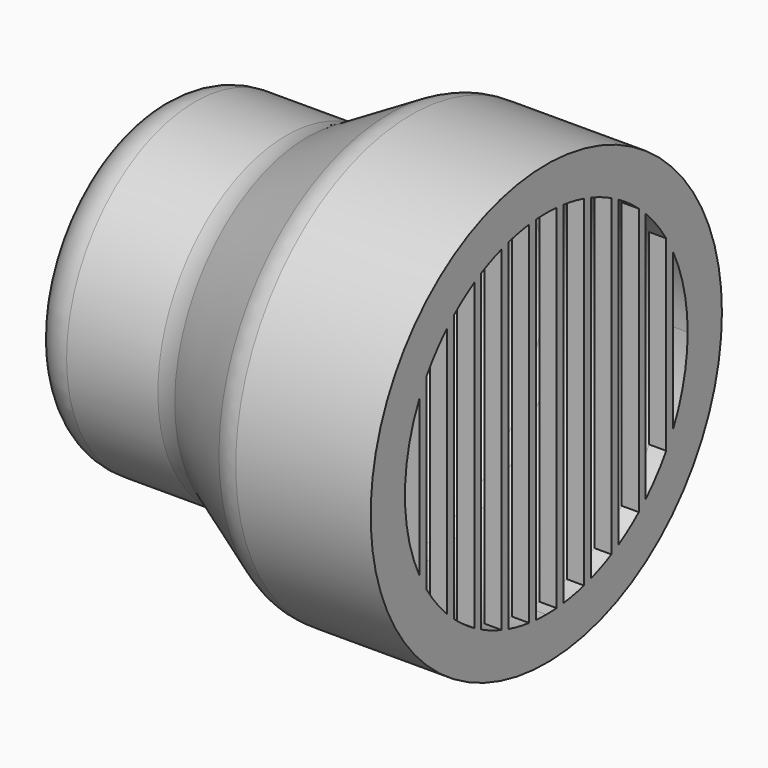
from build123d import *

# Parameters (mm, degrees)
F2_R     = 25.625
F3_DEPTH = 2
F5_DEPTH = 2
F6_R     = 4.99999
F7_R     = 3


# Not quite as in the source:
# - a fillet or chamfer is up to 0.001 mm smaller than in the source, because OpenCascade refuses the exact size


with BuildPart() as f1:
    # F0 (on Top) → F1 (revolve)
    with BuildSketch(Plane.XY):
        Polygon((-18.3333333333, 18.75), (-18.3333333333, 13.75), (0, 13.75), (11.907849302, 20.625), (25.657849302, 20.625), (25.657849302, 25.625), (10.5681033399, 25.625), (-1.3397459622, 18.75), align=None)
    revolve(axis=Axis((-8.7595172226, 0, 0), (1, 0, 0)))

    # F2 (on face) → F3 (join)
    with BuildSketch(Plane.YZ.offset(25.657849302)):
        Circle(F2_R)
    extrude(amount=F3_DEPTH)

    # F4 (on face) → F5 (cut, through all)
    with BuildSketch(Plane.YZ.offset(27.657849302)):
        with BuildLine():
            ThreePointArc((20.625, 0), (20.0867260274, 4.6812458278), (18.5, 9.1181481124))
            Line((18.5, 9.1181481124), (18.5, -9.1181481124))
            ThreePointArc((18.5, -9.1181481124), (20.0867260274, -4.6812458278), (20.625, 0))
        make_face()
        with BuildLine():
            ThreePointArc((17.5, 10.9151557479), (16.1096351924, 12.8790635905), (14.5, 14.6676727875))
            Line((14.5, 14.6676727875), (14.5, -14.6676727875))
            ThreePointArc((14.5, -14.6676727875), (16.1096351924, -12.8790635905), (17.5, -10.9151557479))
            Line((17.5, -10.9151557479), (17.5, 10.9151557479))
        make_face()
        with BuildLine():
            ThreePointArc((13.5, 15.5929671647), (12.0484676296, 16.7399239179), (10.5, 17.7522005678))
            Line((10.5, 17.7522005678), (10.5, -17.7522005678))
            ThreePointArc((10.5, -17.7522005678), (12.0484676296, -16.7399239179), (13.5, -15.5929671647))
            Line((13.5, -15.5929671647), (13.5, 15.5929671647))
        make_face()
        with BuildLine():
            ThreePointArc((9.5, 18.3068463969), (8.0250486473, 18.9997162929), (6.5, 19.573978262))
            Line((6.5, 19.573978262), (6.5, -19.573978262))
            ThreePointArc((6.5, -19.573978262), (8.0250486473, -18.9997162929), (9.5, -18.3068463969))
            Line((9.5, -18.3068463969), (9.5, 18.3068463969))
        make_face()
        with BuildLine():
            ThreePointArc((5.5, 19.8781444054), (4.0110398588, 20.2312180615), (2.5, 20.4729241927))
            Line((2.5, 20.4729241927), (2.5, -20.4729241927))
            ThreePointArc((2.5, -20.4729241927), (4.0110398588, -20.2312180615), (5.5, -19.8781444054))
            Line((5.5, -19.8781444054), (5.5, 19.8781444054))
        make_face()
        with BuildLine():
            ThreePointArc((1.5, 20.5703822279), (0.7504970188, 20.6113410341), (0, 20.625))
            ThreePointArc((0, 20.625), (-0.7504970188, 20.6113410341), (-1.5, 20.5703822279))
            Line((-1.5, 20.5703822279), (-1.5, -20.5703822279))
            ThreePointArc((-1.5, -20.5703822279), (-0.7504970188, -20.6113410341), (0, -20.625))
            ThreePointArc((0, -20.625), (0.7504970188, -20.6113410341), (1.5, -20.5703822279))
            Line((1.5, -20.5703822279), (1.5, 20.5703822279))
        make_face()
        with BuildLine():
            Line((-2.5, -20.4729241927), (-2.5, 20.4729241927))
            ThreePointArc((-2.5, 20.4729241927), (-4.0110398588, 20.2312180615), (-5.5, 19.8781444054))
            Line((-5.5, 19.8781444054), (-5.5, -19.8781444054))
            ThreePointArc((-5.5, -19.8781444054), (-4.0110398588, -20.2312180615), (-2.5, -20.4729241927))
        make_face()
        with BuildLine():
            Line((-6.5, -19.573978262), (-6.5, 19.573978262))
            ThreePointArc((-6.5, 19.573978262), (-8.0250486473, 18.9997162929), (-9.5, 18.3068463969))
            Line((-9.5, 18.3068463969), (-9.5, -18.3068463969))
            ThreePointArc((-9.5, -18.3068463969), (-8.0250486473, -18.9997162929), (-6.5, -19.573978262))
        make_face()
        with BuildLine():
            Line((-10.5, -17.7522005678), (-10.5, 17.7522005678))
            ThreePointArc((-10.5, 17.7522005678), (-12.0484676296, 16.7399239179), (-13.5, 15.5929671647))
            Line((-13.5, 15.5929671647), (-13.5, -15.5929671647))
            ThreePointArc((-13.5, -15.5929671647), (-12.0484676296, -16.7399239179), (-10.5, -17.7522005678))
        make_face()
        with BuildLine():
            Line((-14.5, -14.6676727875), (-14.5, 14.6676727875))
            ThreePointArc((-14.5, 14.6676727875), (-16.1096351924, 12.8790635905), (-17.5, 10.9151557479))
            Line((-17.5, 10.9151557479), (-17.5, -10.9151557479))
            ThreePointArc((-17.5, -10.9151557479), (-16.1096351924, -12.8790635905), (-14.5, -14.6676727875))
        make_face()
        with BuildLine():
            Line((-18.5, -9.1181481124), (-18.5, 9.1181481124))
            ThreePointArc((-18.5, 9.1181481124), (-20.625, 0), (-18.5, -9.1181481124))
        make_face()
    extrude(amount=-F5_DEPTH, mode=Mode.SUBTRACT)

    # F6 (radius 5 in the source; OpenCascade refuses exactly that, so slightly less here)
    f6_edges = [f1.edges().sort_by_distance(p)[0] for p in [
        (-18.333333, -18.75, 0),
        (-1.339746, -18.75, 0),
        (10.568103, -25.625, 0),
    ]]
    fillet(f6_edges, radius=F6_R)

    # F7
    f7_edges = [f1.edges().sort_by_distance(p)[0] for p in [
        (11.907849, -20.625, 0),
        (0, -13.75, 0),
    ]]
    fillet(f7_edges, radius=F7_R)


solid = f1.part
